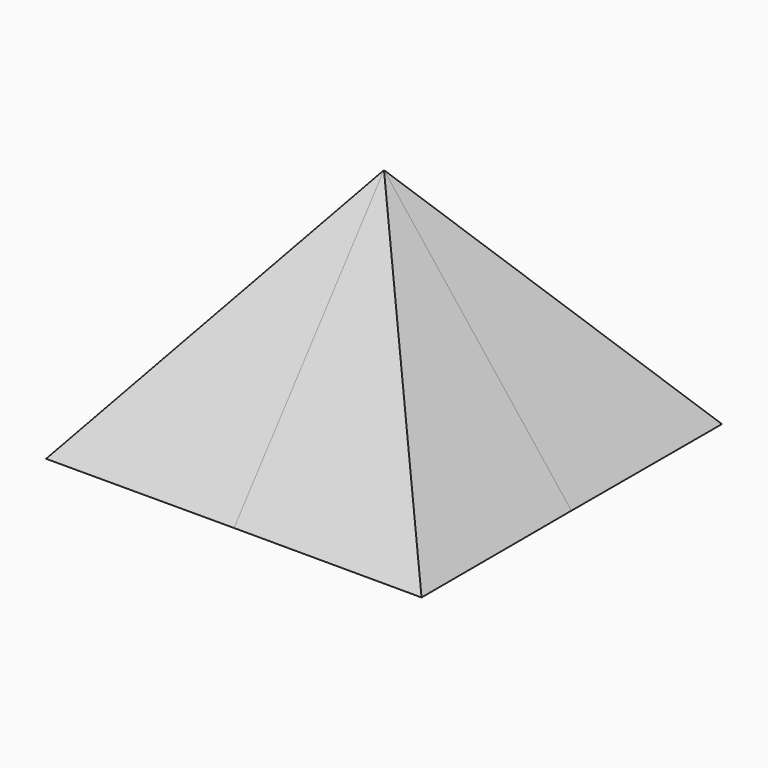
from build123d import *


# Not quite as in the source:
# - a feature of the source that left no trace in its solid (it failed there, or was rolled back) is left out


with BuildPart() as f3:
    # F2 (on offset) → F3 section 0
    with BuildSketch(Plane.XY.offset(146)):
        Polygon((0.4598601322, 0), (0.4605799133, 0.4605799133), (0, 0.4598601322), (-0.4605799133, 0.4605799133), (-0.4598601322, 0), (-0.4605799133, -0.4605799133), (0, -0.4598601322), (0.4605799133, -0.4605799133), align=None)
    # F0 (on Top) → F3 section 1
    with BuildSketch(Plane.XY):
        Polygon((0, 115), (-115.18, 115.18), (-115, 0), (-115.18, -115.18), (0, -115), (115.18, -115.18), (115, 0), (115.18, 115.18), align=None)
    loft()


solid = f3.part
